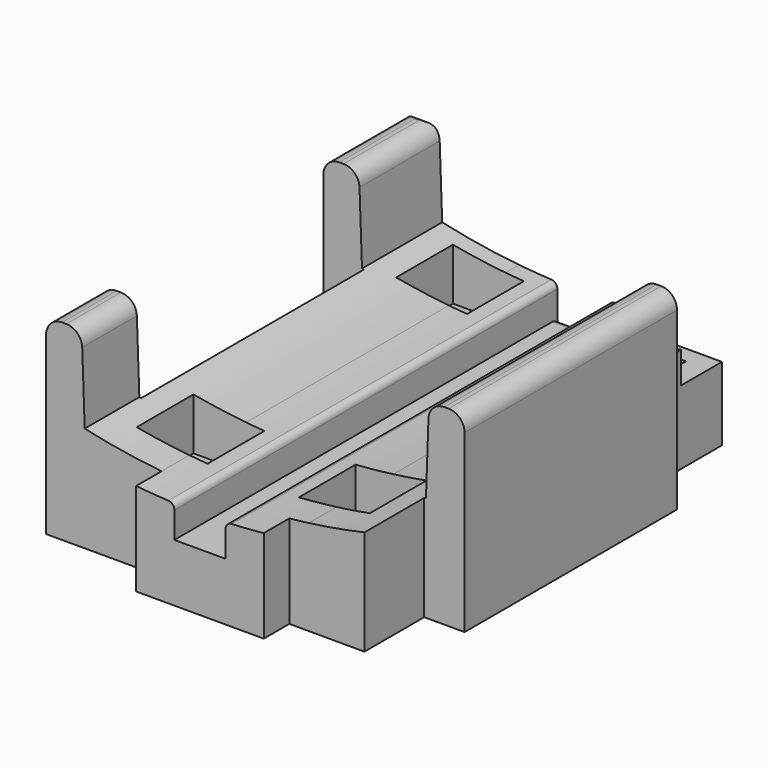
from build123d import *

# Parameters (mm, degrees)
F1_DEPTH     = 75
F3_START     = -67
F3_DEPTH     = 8
F4_D         = 6.7564
F5_START     = -7.6
F2_W         = 5.5565
F2_H         = 5.5565
F5_DEPTH     = 22.401
F2_W_2       = 6.328
F2_H_2       = 8.3
F2_H_3       = 43.6
F2_H_4       = 8.4
F2_H_5       = 16.7
F2_H_6       = 0.7
F6_DEPTH     = 30
F7_R         = 1
F8_DEPTH     = 5
F9_T1_DEPTH  = 23.2
F9_T3_DEPTH  = 22.7686226101
F9_T5_DEPTH  = 27.2
F9_T7_DEPTH  = 26.7686226101
F9_T9_DEPTH  = 53.6686226101
F9_T11_DEPTH = 54.1


# Not quite as in the source:
# - a fillet or chamfer that OpenCascade refuses, or shapes differently, is made with other operations: its cross-section is extruded or revolved along the edge and cut away or added
# - a feature names something its author has since deleted; it is built from what else it names


with BuildPart() as f1:
    # F0 (on Front) → F1 (new body)
    with BuildSketch(Plane.XZ):
        with BuildLine():
            Line((-25, -84.153), (-25, -96.9278597721))
            ThreePointArc((-25, -96.9278597721), (-23.5277037783, -97.2957201264), (-22.05, -97.6412182431))
            Line((-22.05, -97.6412182431), (-22.5238, -84.153))
            Line((-22.5238, -84.153), (-25, -84.153))
        make_face()
        with BuildLine():
            ThreePointArc((22.05, -97.6412182431), (23.5277037782, -97.2957201264), (25, -96.9278597721))
            Line((25, -96.9278597721), (25, -84.153))
            Line((25, -84.153), (22.5238, -84.153))
            Line((22.5238, -84.153), (22.05, -97.6412182431))
        make_face()
        with BuildLine():
            Line((22.05, -102.6412182431), (22.05, -97.6412182431))
            ThreePointArc((22.05, -97.6412182431), (17.5683261722, -98.5462526711), (13.05, -99.2456926017))
            Line((13.05, -99.2456926017), (13.05, -102.6412182431))
            Line((13.05, -102.6412182431), (22.05, -102.6412182431))
        make_face()
        with BuildLine():
            ThreePointArc((-4, -100.0200479904), (-7.0031613127, -99.8547231313), (-10, -99.5992469851))
            Line((-10, -99.5992469851), (-10, -114.153))
            Line((-10, -114.153), (0, -114.153))
            Line((0, -114.153), (10, -114.153))
            Line((10, -114.153), (10, -99.5992469851))
            ThreePointArc((10, -99.5992469851), (7.0031613127, -99.8547231313), (4, -100.0200479904))
            Line((4, -100.0200479904), (4, -105.0902182431))
            Line((4, -105.0902182431), (-4, -105.0902182431))
            Line((-4, -105.0902182431), (-4, -100.0200479904))
        make_face()
        with BuildLine():
            ThreePointArc((-25, -96.9278597721), (-26.5533240856, -96.5138900884), (-28.0998, -96.0750292217))
            Line((-28.0998, -96.0750292217), (-28.0998, -104.153))
            Line((-28.0998, -104.153), (-28.0998, -114.153))
            Line((-28.0998, -114.153), (-25, -114.153))
            Line((-25, -114.153), (-25, -96.9278597721))
        make_face()
        with BuildLine():
            Line((28.0998, -104.153), (28.0998, -96.0750292217))
            ThreePointArc((28.0998, -96.0750292217), (26.5533240856, -96.5138900884), (25, -96.9278597721))
            Line((25, -96.9278597721), (25, -114.153))
            Line((25, -114.153), (28.0998, -114.153))
            Line((28.0998, -114.153), (28.0998, -104.153))
        make_face()
        with BuildLine():
            ThreePointArc((25, -96.9278597721), (26.5533240856, -96.5138900884), (28.0998, -96.0750292217))
            Line((28.0998, -96.0750292217), (28.0998, -84.153))
            Line((28.0998, -84.153), (25, -84.153))
            Line((25, -84.153), (25, -96.9278597721))
        make_face()
        with BuildLine():
            Line((-28.0998, -84.153), (-28.0998, -96.0750292217))
            ThreePointArc((-28.0998, -96.0750292217), (-26.5533240856, -96.5138900884), (-25, -96.9278597721))
            Line((-25, -96.9278597721), (-25, -84.153))
            Line((-25, -84.153), (-28.0998, -84.153))
        make_face()
        with BuildLine():
            Line((25, -114.153), (25, -96.9278597721))
            ThreePointArc((25, -96.9278597721), (23.5277037782, -97.2957201264), (22.05, -97.6412182431))
            Line((22.05, -97.6412182431), (22.05, -102.6412182431))
            Line((22.05, -102.6412182431), (13.05, -102.6412182431))
            Line((13.05, -102.6412182431), (13.05, -99.2456926017))
            ThreePointArc((13.05, -99.2456926017), (11.5263556763, -99.4341647766), (10, -99.5992469851))
            Line((10, -99.5992469851), (10, -114.153))
            Line((10, -114.153), (22.5238, -114.153))
            Line((22.5238, -114.153), (25, -114.153))
        make_face()
        with BuildLine():
            ThreePointArc((-22.05, -97.6412182431), (-23.5277037783, -97.2957201264), (-25, -96.9278597721))
            Line((-25, -96.9278597721), (-25, -114.153))
            Line((-25, -114.153), (-22.5238, -114.153))
            Line((-22.5238, -114.153), (-10, -114.153))
            Line((-10, -114.153), (-10, -99.5992469851))
            ThreePointArc((-10, -99.5992469851), (-16.0548775809, -98.8041036894), (-22.05, -97.6412182431))
        make_face()
    extrude(amount=-F1_DEPTH)

    # F0 (on Front) → F3 (cut)
    with BuildSketch(Plane.XZ.offset(F3_START)):
        with BuildLine():
            Line((22.05, -102.6412182431), (22.05, -97.6412182431))
            ThreePointArc((22.05, -97.6412182431), (17.5683261722, -98.5462526711), (13.05, -99.2456926017))
            Line((13.05, -99.2456926017), (13.05, -102.6412182431))
            Line((13.05, -102.6412182431), (22.05, -102.6412182431))
        make_face()
    extrude(amount=-F3_DEPTH, mode=Mode.SUBTRACT)

    # F4 (through all)
    with Locations(Plane(origin=(0, 0, -114.153), x_dir=(1, 0, 0), z_dir=(0, 0, -1))):
        with Locations((-12.7, -168.4), (12.7, -168.4), (-12.7, -117.6), (12.7, -117.6), (-12.7, -66.8), (12.7, -66.8), (-12.7, -16), (12.7, -16)):
            Hole(F4_D / 2)

    # F2 (on face) → F5 (cut)
    with BuildSketch(Plane(origin=(0, 0, -114.153), x_dir=(1, 0, 0), z_dir=(0, 0, -1)).offset(F5_START)):
        Polygon((-12.7, -173.9565), (-12.7, -168.4), (-12.7, -162.8435), (-18.2565, -162.8435), (-18.2565, -173.9565), align=None)
        with Locations((-9.92175, -165.62175)):
            Rectangle(F2_W, F2_H)
        with Locations((-9.92175, -171.17825)):
            Rectangle(F2_W, F2_H)
        with Locations((9.92175, -171.17825)):
            Rectangle(F2_W, F2_H)
        with Locations((9.92175, -165.62175)):
            Rectangle(F2_W, F2_H)
        Polygon((12.7, -162.8435), (12.7, -168.4), (12.7, -173.9565), (18.2565, -173.9565), (18.2565, -162.8435), align=None)
        Polygon((18.2565, -112.0435), (12.7, -112.0435), (12.7, -117.6), (12.7, -123.1565), (18.2565, -123.1565), align=None)
        with Locations((9.92175, -114.82175)):
            Rectangle(F2_W, F2_H)
        with Locations((9.92175, -120.37825)):
            Rectangle(F2_W, F2_H)
        with Locations((-9.92175, -120.37825)):
            Rectangle(F2_W, F2_H)
        with Locations((-9.92175, -114.82175)):
            Rectangle(F2_W, F2_H)
        Polygon((-12.7, -117.6), (-12.7, -112.0435), (-18.2565, -112.0435), (-18.2565, -123.1565), (-12.7, -123.1565), align=None)
        with Locations((-9.92175, -64.02175)):
            Rectangle(F2_W, F2_H)
        with Locations((-9.92175, -69.57825)):
            Rectangle(F2_W, F2_H)
        Polygon((-12.7, -72.3565), (-12.7, -66.8), (-12.7, -61.2435), (-18.2565, -61.2435), (-18.2565, -72.3565), align=None)
        with Locations((9.92175, -64.02175)):
            Rectangle(F2_W, F2_H)
        with Locations((9.92175, -69.57825)):
            Rectangle(F2_W, F2_H)
        Polygon((12.7, -61.2435), (12.7, -66.8), (12.7, -72.3565), (18.2565, -72.3565), (18.2565, -61.2435), align=None)
        with Locations((9.92175, -18.77825)):
            Rectangle(F2_W, F2_H)
        with Locations((9.92175, -13.22175)):
            Rectangle(F2_W, F2_H)
        Polygon((18.2565, -10.4435), (12.7, -10.4435), (12.7, -16), (12.7, -21.5565), (18.2565, -21.5565), align=None)
        with Locations((-9.92175, -13.22175)):
            Rectangle(F2_W, F2_H)
        Polygon((-12.7, -16), (-12.7, -10.4435), (-18.2565, -10.4435), (-18.2565, -21.5565), (-12.7, -21.5565), align=None)
        with Locations((-9.92175, -18.77825)):
            Rectangle(F2_W, F2_H)
    extrude(amount=-F5_DEPTH, mode=Mode.SUBTRACT)

    # F2 (on face) → F6 (cut, through all)
    with BuildSketch(Plane(origin=(0, 0, -114.153), x_dir=(1, 0, 0), z_dir=(0, 0, -1))):
        with Locations((24.9358, -70.85)):
            Rectangle(F2_W_2, F2_H_2)
        with Locations((-24.9358, -37.5)):
            Rectangle(F2_W_2, F2_H_3)
        with Locations((24.9358, -62.5)):
            Rectangle(F2_W_2, F2_H_4)
        with Locations((24.9358, -8.35)):
            Rectangle(F2_W_2, F2_H_5)
        with Locations((24.9358, 0.35)):
            Rectangle(F2_W_2, F2_H_6)
    extrude(amount=-F6_DEPTH, mode=Mode.SUBTRACT)

    # F7
    f7_edges = [f1.edges().sort_by_distance(p)[0] for p in [
        (-28.0998, 75, -99.153),
        (-4, 37.5, -100.020048),
        (4, 37.5, -100.020048),
        (0, 75, -105.090218),
        (-25.3118, 75, -84.153),
    ]]
    fillet(f7_edges, radius=F7_R)

    # F0 (on Front) → F8 (cut)
    with BuildSketch(Plane.XZ):
        with BuildLine():
            ThreePointArc((-22.05, -97.6412182431), (-23.5277037783, -97.2957201264), (-25, -96.9278597721))
            Line((-25, -96.9278597721), (-25, -114.153))
            Line((-25, -114.153), (-22.5238, -114.153))
            Line((-22.5238, -114.153), (-10, -114.153))
            Line((-10, -114.153), (-10, -99.5992469851))
            ThreePointArc((-10, -99.5992469851), (-16.0548775809, -98.8041036894), (-22.05, -97.6412182431))
        make_face()
        with BuildLine():
            Line((25, -114.153), (25, -96.9278597721))
            ThreePointArc((25, -96.9278597721), (23.5277037782, -97.2957201264), (22.05, -97.6412182431))
            Line((22.05, -97.6412182431), (22.05, -102.6412182431))
            Line((22.05, -102.6412182431), (13.05, -102.6412182431))
            Line((13.05, -102.6412182431), (13.05, -99.2456926017))
            ThreePointArc((13.05, -99.2456926017), (11.5263556763, -99.4341647766), (10, -99.5992469851))
            Line((10, -99.5992469851), (10, -114.153))
            Line((10, -114.153), (22.5238, -114.153))
            Line((22.5238, -114.153), (25, -114.153))
        make_face()
        with BuildLine():
            Line((22.05, -102.6412182431), (22.05, -97.6412182431))
            ThreePointArc((22.05, -97.6412182431), (17.5683261722, -98.5462526711), (13.05, -99.2456926017))
            Line((13.05, -99.2456926017), (13.05, -102.6412182431))
            Line((13.05, -102.6412182431), (22.05, -102.6412182431))
        make_face()
        with BuildLine():
            ThreePointArc((-25, -96.9278597721), (-26.5533240856, -96.5138900884), (-28.0998, -96.0750292217))
            Line((-28.0998, -96.0750292217), (-28.0998, -104.153))
            Line((-28.0998, -104.153), (-28.0998, -114.153))
            Line((-28.0998, -114.153), (-25, -114.153))
            Line((-25, -114.153), (-25, -96.9278597721))
        make_face()
        with BuildLine():
            Line((-28.0998, -84.153), (-28.0998, -96.0750292217))
            ThreePointArc((-28.0998, -96.0750292217), (-26.5533240856, -96.5138900884), (-25, -96.9278597721))
            Line((-25, -96.9278597721), (-25, -84.153))
            Line((-25, -84.153), (-28.0998, -84.153))
        make_face()
        with BuildLine():
            Line((-25, -84.153), (-25, -96.9278597721))
            ThreePointArc((-25, -96.9278597721), (-23.5277037783, -97.2957201264), (-22.05, -97.6412182431))
            Line((-22.05, -97.6412182431), (-22.5238, -84.153))
            Line((-22.5238, -84.153), (-25, -84.153))
        make_face()
    extrude(amount=-F8_DEPTH, mode=Mode.SUBTRACT)

    # F9: fillet of radius 2.5 on 6 edges, made by hand

    # F9_s2 → F9_t1 (cut)
    with BuildSketch(Plane.XZ.offset(-21.95)):
        with BuildLine():
            ThreePointArc((-25.5998, -84.153), (-27.367566953, -84.885233047), (-28.0998, -86.653))
            Line((-28.0998, -86.653), (-28.0998, -84.153))
            Line((-28.0998, -84.153), (-25.5998, -84.153))
        make_face()
    extrude(amount=F9_T1_DEPTH, mode=Mode.SUBTRACT)

    # F9_s4 → F9_t3 (cut)
    with BuildSketch(Plane.XZ.offset(-21.7343113051)):
        with BuildLine():
            ThreePointArc((-24.937524522, -84.153), (-23.2010637724, -84.8544716947), (-22.4390654746, -86.565236748))
            Line((-22.4390654746, -86.565236748), (-22.5238, -84.153))
            Line((-22.5238, -84.153), (-24.937524522, -84.153))
        make_face()
    extrude(amount=F9_T3_DEPTH, mode=Mode.SUBTRACT)

    # F9_s6 → F9_t5 (cut)
    with BuildSketch(Plane.XZ.offset(-80.25)):
        with BuildLine():
            ThreePointArc((-28.0998, -86.653), (-27.367566953, -84.885233047), (-25.5998, -84.153))
            Line((-25.5998, -84.153), (-28.0998, -84.153))
            Line((-28.0998, -84.153), (-28.0998, -86.653))
        make_face()
    extrude(amount=F9_T5_DEPTH, mode=Mode.SUBTRACT)

    # F9_s8 → F9_t7 (cut)
    with BuildSketch(Plane.XZ.offset(-80.0343113051)):
        with BuildLine():
            ThreePointArc((-24.937524522, -84.153), (-23.2010637724, -84.8544716947), (-22.4390654746, -86.565236748))
            Line((-22.4390654746, -86.565236748), (-22.5238, -84.153))
            Line((-22.5238, -84.153), (-24.937524522, -84.153))
        make_face()
    extrude(amount=F9_T7_DEPTH, mode=Mode.SUBTRACT)

    # F9_s10 → F9_t9 (cut)
    with BuildSketch(Plane.XZ.offset(-64.3343113051)):
        with BuildLine():
            ThreePointArc((24.937524522, -84.153), (23.2010637724, -84.8544716947), (22.4390654746, -86.565236748))
            Line((22.4390654746, -86.565236748), (22.5238, -84.153))
            Line((22.5238, -84.153), (24.937524522, -84.153))
        make_face()
    extrude(amount=F9_T9_DEPTH, mode=Mode.SUBTRACT)

    # F9_s12 → F9_t11 (cut)
    with BuildSketch(Plane.XZ.offset(-64.55)):
        with BuildLine():
            ThreePointArc((28.0998, -86.653), (27.367566953, -84.885233047), (25.5998, -84.153))
            Line((25.5998, -84.153), (28.0998, -84.153))
            Line((28.0998, -84.153), (28.0998, -86.653))
        make_face()
    extrude(amount=F9_T11_DEPTH, mode=Mode.SUBTRACT)


solid = f1.part
